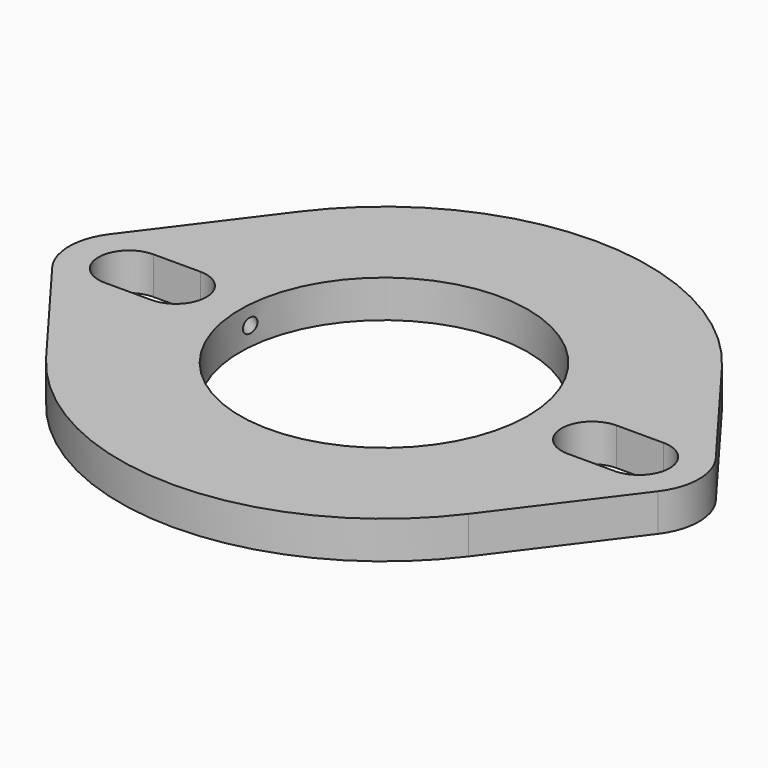
from build123d import *

# Parameters (mm, degrees)
F0_R     = 30.48
F1_DEPTH = 7.9375
F2_R     = 1.5
F3_DEPTH = 32.0605350826


# Not quite as in the source:
# - a length typed as a fraction of an inch, garbled in the dataset ("3 / 203.2 mm" for 3/8 in), is restored


with BuildPart() as f1:
    # F0 (on Top) → F1 (new body)
    with BuildSketch(Plane.XY):
        with BuildLine():
            Line((-64.135, -7.62), (-44.704, -33.528))
            ThreePointArc((-44.704, -33.528), (0, -55.88), (44.704, -33.528))
            Line((44.704, -33.528), (64.135, -7.62))
            ThreePointArc((64.135, -7.62), (66.675, 0), (64.135, 7.62))
            Line((64.135, 7.62), (44.704, 33.528))
            ThreePointArc((44.704, 33.528), (0, 55.88), (-44.704, 33.528))
            Line((-44.704, 33.528), (-64.135, 7.62))
            ThreePointArc((-64.135, 7.62), (-66.675, 0), (-64.135, -7.62))
        make_face()
        with BuildLine():
            ThreePointArc((-53.975, -6.477), (-60.452, 0), (-53.975, 6.477))
            Line((-53.975, 6.477), (-44.069, 6.477))
            ThreePointArc((-44.069, 6.477), (-37.592, 0), (-44.069, -6.477))
            Line((-44.069, -6.477), (-53.975, -6.477))
        make_face(mode=Mode.SUBTRACT)
        Circle(F0_R, mode=Mode.SUBTRACT)
        with BuildLine():
            ThreePointArc((44.069, -6.477), (37.592, 0), (44.069, 6.477))
            Line((44.069, 6.477), (53.9750001618, 6.477))
            ThreePointArc((53.9750001618, 6.477), (60.452, -8.09e-08), (53.975, -6.477))
            Line((53.975, -6.477), (44.069, -6.477))
        make_face(mode=Mode.SUBTRACT)
    extrude(amount=F1_DEPTH)

    # F2 (on face) → F3 (cut, up to face)
    with BuildSketch(Plane(origin=(-44.704, 33.528, 0), x_dir=(-0.6, -0.8, 0), z_dir=(-0.8, 0.6, 0))):
        with Locations((16.1925, 3.96875)):
            Circle(F2_R)
    extrude(amount=-F3_DEPTH, mode=Mode.SUBTRACT)


solid = f1.part
